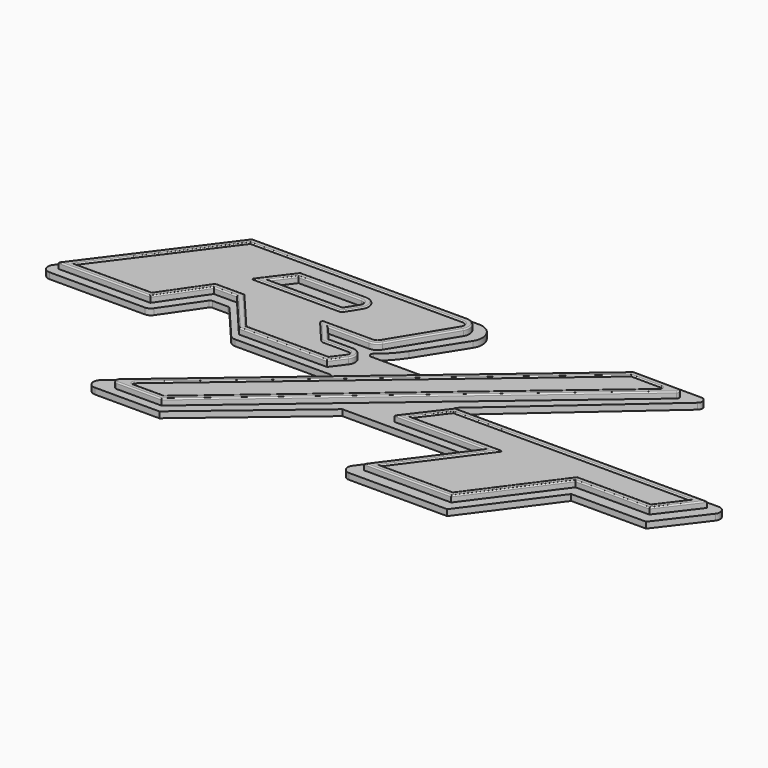
from build123d import *

# Parameters (mm, degrees)
F1_DEPTH = 2.54
F3_DEPTH = 2.54
F5_DEPTH = 2.54
F9_DEPTH = 0.508
F7_R     = 0.50799


# Not quite as in the source:
# - a fillet or chamfer is up to 0.001 mm smaller than in the source, because OpenCascade refuses the exact size


with BuildPart() as f1:
    # F0 (on Top) → F1 (new body)
    with BuildSketch(Plane.XY):
        with BuildLine():
            ThreePointArc((-245.2867057585, 196.0372725906), (-245.8553406914, 195.9028580401), (-246.303608996, 195.5280667845))
            Line((-246.303608996, 195.5280667845), (-286.1584039652, 142.2568005721))
            ThreePointArc((-286.1584039652, 142.2568005721), (-286.4332926298, 139.1776112706), (-283.8030790316, 137.5531276726))
            Line((-283.8030790316, 137.5531276726), (-244.1552884223, 137.5531276726))
            ThreePointArc((-244.1552884223, 137.5531276726), (-242.676229187, 137.9186777658), (-241.5377496314, 138.9311536388))
            Line((-241.5377496314, 138.9311536388), (-230.9500368786, 154.3536073393))
            ThreePointArc((-230.9500368786, 154.3536073393), (-230.4946450563, 154.7585976885), (-229.9030213622, 154.9048177258))
            Line((-229.9030213622, 154.9048177258), (-223.4319893817, 154.9048177258))
            ThreePointArc((-223.4319893817, 154.9048177258), (-222.8981310818, 154.7871611276), (-222.463189241, 154.4559914512))
            Line((-222.463189241, 154.4559914512), (-209.7825220275, 139.4956586958))
            ThreePointArc((-209.7825220275, 139.4956586958), (-208.6951674254, 138.6677345048), (-207.3605216756, 138.3735930092))
            Line((-207.3605216756, 138.3735930092), (-167.7892972517, 138.3735930092))
            ThreePointArc((-167.7892972517, 138.3735930092), (-166.9553293934, 137.7925193173), (-167.2115680195, 136.8089082201))
            Line((-167.2115680195, 136.8089082201), (-223.5524593467, 88.6358837388))
            ThreePointArc((-223.5524593467, 88.6358837388), (-224.401761015, 85.3757095864), (-221.6375786431, 83.4497436876))
            Line((-221.6375786431, 83.4497436876), (-194.8649699805, 83.4497436876))
            Line((-194.8649699805, 83.4497436876), (-149.4059527633, 121.7579135561))
            Line((-149.4059527633, 121.7579135561), (-100.5507462578, 121.7579135561))
            Line((-100.5507462578, 121.7579135561), (-121.9878317389, 92.7682602457))
            ThreePointArc((-121.9878317389, 92.7682602457), (-122.2464609413, 89.7274503693), (-119.6477423423, 88.1274268031))
            Line((-119.6477423423, 88.1274268031), (-78.8742303848, 88.1274268031))
            Line((-78.8742303848, 88.1274268031), (-54.1144270955, 121.6104352103))
            Line((-54.1144270955, 121.6104352103), (-22.9366910897, 121.6104352103))
            Line((-22.9366910897, 121.6104352103), (-8.9016964649, 140.0485662822))
            ThreePointArc((-8.9016964649, 140.0485662822), (-8.6207642896, 142.9884064855), (-11.130164208, 144.5454855965))
            Line((-11.130164208, 144.5454855965), (-120.6925099216, 144.5454855965))
            ThreePointArc((-120.6925099216, 144.5454855965), (-121.2867775914, 144.9567202359), (-121.1113336048, 145.6577818592))
            Line((-121.1113336048, 145.6577818592), (-62.1562381195, 197.3904103448))
            ThreePointArc((-62.1562381195, 197.3904103448), (-61.583083752, 199.680694207), (-63.5244846344, 201.0241482302))
            Line((-63.5244846344, 201.0241482302), (-91.5325754885, 201.0241482302))
            Line((-91.5325754885, 201.0241482302), (-144.0581907195, 156.390979886))
            Line((-144.0581907195, 156.390979886), (-165.1567965746, 156.390979886))
            ThreePointArc((-165.1567965746, 156.390979886), (-166.2861296508, 157.2759629471), (-165.8412963152, 158.6400419474))
            ThreePointArc((-165.8412963152, 158.6400419474), (-161.5040417608, 162.5655921163), (-157.946344878, 167.2093528863))
            Line((-157.946344878, 167.2093528863), (-146.2688178366, 185.7109197082))
            ThreePointArc((-146.2688178366, 185.7109197082), (-146.0663995706, 192.5553078333), (-151.9623764525, 196.0372725906))
            Line((-151.9623764525, 196.0372725906), (-245.2867057585, 196.0372725906))
        make_face()
    extrude(amount=F1_DEPTH)

    # F2 (on face) → F3 (join)
    with BuildSketch(Plane.XY.offset(2.54)):
        with BuildLine():
            Line((-75.6383077882, 195.1749867248), (-88.1063342094, 195.2720095674))
            Line((-88.1063342094, 195.2720095674), (-211.0118440568, 90.8230394157))
            ThreePointArc((-211.0118440568, 90.8230394157), (-211.2321021719, 89.9853005359), (-210.5217670945, 89.4895746581))
            Line((-210.5217670945, 89.4895746581), (-197.7361927904, 89.4895746581))
            Line((-197.7361927904, 89.4895746581), (-75.1047645055, 193.7056216727))
            ThreePointArc((-75.1047645055, 193.7056216727), (-74.860941222, 194.6257070651), (-75.6383077882, 195.1749867248))
        make_face()
        Polygon((-18.5225492173, 139.0465293437), (-117.1023442206, 139.0465293437), (-125.6702630111, 127.7906354944), (-87.9282544571, 127.7906354944), (-112.1474074595, 95.0387555978), (-82.0121606334, 95.0387555978), (-57.1953153693, 128.5989026195), (-26.475219927, 128.5989026195), align=None)
        with BuildLine():
            Line((-154.6691002865, 190.8006613512), (-242.8746338045, 190.8006613512))
            Line((-242.8746338045, 190.8006613512), (-278.1461511696, 143.655558918))
            Line((-278.1461511696, 143.655558918), (-246.0618317127, 143.655558918))
            Line((-246.0618317127, 143.655558918), (-233.8889765025, 161.3869897064))
            Line((-233.8889765025, 161.3869897064), (-221.8132032306, 161.3869897064))
            Line((-221.8132032306, 161.3869897064), (-207.2979211807, 144.2622244358))
            Line((-207.2979211807, 144.2622244358), (-173.0524588328, 144.2622244358))
            Line((-173.0524588328, 144.2622244358), (-169.4335754667, 149.0993462762))
            ThreePointArc((-169.4335754667, 149.0993462762), (-169.2980659943, 150.6172674254), (-170.5946594988, 151.4180749655))
            Line((-170.5946594988, 151.4180749655), (-180.6847838701, 151.4180749655))
            ThreePointArc((-180.6847838701, 151.4180749655), (-181.7775167216, 151.6589014734), (-182.6677814942, 152.3367592212))
            Line((-182.6677814942, 152.3367592212), (-190.4167001347, 161.4787388509))
            ThreePointArc((-190.4167001347, 161.4787388509), (-190.5341831318, 162.3460723754), (-189.7965872333, 162.8172644678))
            Line((-189.7965872333, 162.8172644678), (-169.2928134558, 162.8172644678))
            ThreePointArc((-169.2928134558, 162.8172644678), (-168.2285718133, 163.0956607735), (-167.4369771006, 163.8595276385))
            Line((-167.4369771006, 163.8595276385), (-152.9175816859, 187.6819366499))
            ThreePointArc((-152.9175816859, 187.6819366499), (-152.8806469623, 189.7538804922), (-154.6691002865, 190.8006613512))
        make_face()
        with BuildLine():
            Line((-226.7749905586, 171.6903150082), (-217.0877456665, 184.534072876))
            Line((-217.0877456665, 184.534072876), (-189.6498650312, 184.534072876))
            ThreePointArc((-189.6498650312, 184.534072876), (-185.7910307303, 182.2551757043), (-185.9235106507, 177.7756195264))
            Line((-185.9235106507, 177.7756195264), (-189.3198400657, 172.3945644967))
            ThreePointArc((-189.3198400657, 172.3945644967), (-189.8678435628, 171.8780436065), (-190.5971306368, 171.6903150082))
            Line((-190.5971306368, 171.6903150082), (-226.7749905586, 171.6903150082))
        make_face(mode=Mode.SUBTRACT)
    extrude(amount=F3_DEPTH)

    # F4 (on face) → F5 (join)
    with BuildSketch(Plane.XY.offset(2.54)):
        with BuildLine():
            Line((-70.206199124, 197.5622259258), (-88.9910170645, 197.7084043484))
            Line((-88.9910170645, 197.7084043484), (-216.3343642699, 89.4880203493))
            ThreePointArc((-216.3343642699, 89.4880203493), (-216.7353953667, 87.962721989), (-215.4420652433, 87.0601377988))
            Line((-215.4420652433, 87.0601377988), (-196.8433225219, 87.0601377988))
            Line((-196.8433225219, 87.0601377988), (-69.4065238131, 195.3599398264))
            ThreePointArc((-69.4065238131, 195.3599398264), (-69.0410811838, 196.7389649142), (-70.206199124, 197.5622259258))
        make_face()
        Polygon((-118.3068796381, 141.4772123098), (-130.5752409768, 125.3599525283), (-92.748751834, 125.3599525283), (-116.9679048364, 92.6080726317), (-80.7865153898, 92.6080726317), (-55.9696701257, 126.1682196534), (-25.2706845095, 126.1682196534), (-13.6175712516, 141.4772123098), align=None)
        with BuildLine():
            Line((-154.6691002865, 193.2390613512), (-244.0956422463, 193.2390613512))
            Line((-244.0956422463, 193.2390613512), (-283.0157281162, 141.217158918))
            Line((-283.0157281162, 141.217158918), (-244.7781149145, 141.217158918))
            Line((-244.7781149145, 141.217158918), (-232.6052597042, 158.9485897064))
            Line((-232.6052597042, 158.9485897064), (-222.9428665553, 158.9485897064))
            Line((-222.9428665553, 158.9485897064), (-208.4275845055, 141.8238244358))
            Line((-208.4275845055, 141.8238244358), (-171.831450391, 141.8238244358))
            Line((-171.831450391, 141.8238244358), (-167.4811212506, 147.638621424))
            ThreePointArc((-167.4811212506, 147.638621424), (-167.1177419312, 151.7090464965), (-170.5946594988, 153.8564749655))
            Line((-170.5946594988, 153.8564749655), (-180.6847838701, 153.8564749655))
            ThreePointArc((-180.6847838701, 153.8564749655), (-180.7525087857, 153.8714008048), (-180.807685224, 153.9134127739))
            Line((-180.807685224, 153.9134127739), (-186.2879270512, 160.3788644678))
            Line((-186.2879270512, 160.3788644678), (-169.2928134558, 160.3788644678))
            ThreePointArc((-169.2928134558, 160.3788644678), (-167.0345504492, 160.9696063194), (-165.3548294304, 162.5904903501))
            Line((-165.3548294304, 162.5904903501), (-150.8354340157, 186.4128993614))
            ThreePointArc((-150.8354340157, 186.4128993614), (-150.7545925081, 190.9479018563), (-154.6691002865, 193.2390613512))
        make_face()
        with BuildLine():
            Line((-221.8816466958, 174.1287150082), (-215.872667649, 182.095672876))
            Line((-215.872667649, 182.095672876), (-189.6498650312, 182.095672876))
            ThreePointArc((-189.6498650312, 182.095672876), (-187.9263663476, 181.0778327799), (-187.9855367992, 179.0770966575))
            Line((-187.9855367992, 179.0770966575), (-191.1087782565, 174.1287150082))
            Line((-191.1087782565, 174.1287150082), (-221.8816466958, 174.1287150082))
        make_face(mode=Mode.SUBTRACT)
    extrude(amount=F5_DEPTH)

    # F6 (on face) → F9 (cut)
    with BuildSketch(Plane.XY.offset(5.08)):
        with BuildLine():
            ThreePointArc((-190.4167001347, 161.4787388509), (-190.5341831318, 162.3460723754), (-189.7965872333, 162.8172644678))
            Line((-189.7965872333, 162.8172644678), (-169.2928134558, 162.8172644678))
            ThreePointArc((-169.2928134558, 162.8172644678), (-168.2285718133, 163.0956607735), (-167.4369771006, 163.8595276385))
            Line((-167.4369771006, 163.8595276385), (-152.9175816859, 187.6819366499))
            ThreePointArc((-152.9175816859, 187.6819366499), (-152.8806469623, 189.7538804922), (-154.6691002865, 190.8006613512))
            Line((-154.6691002865, 190.8006613512), (-242.8746338045, 190.8006613512))
            Line((-242.8746338045, 190.8006613512), (-278.1461511696, 143.655558918))
            Line((-278.1461511696, 143.655558918), (-246.0618317127, 143.655558918))
            Line((-246.0618317127, 143.655558918), (-233.8889765025, 161.3869897064))
            Line((-233.8889765025, 161.3869897064), (-221.8132032306, 161.3869897064))
            Line((-221.8132032306, 161.3869897064), (-207.2979211807, 144.2622244358))
            Line((-207.2979211807, 144.2622244358), (-173.0524588328, 144.2622244358))
            Line((-173.0524588328, 144.2622244358), (-169.4335754667, 149.0993462762))
            ThreePointArc((-169.4335754667, 149.0993462762), (-169.2980659943, 150.6172674254), (-170.5946594988, 151.4180749655))
            Line((-170.5946594988, 151.4180749655), (-180.6847838701, 151.4180749655))
            ThreePointArc((-180.6847838701, 151.4180749655), (-181.7775167216, 151.6589014734), (-182.6677814942, 152.3367592212))
            Line((-182.6677814942, 152.3367592212), (-190.4167001347, 161.4787388509))
        make_face()
        with BuildLine():
            Line((-226.7749905586, 171.6903150082), (-217.0877456665, 184.534072876))
            Line((-217.0877456665, 184.534072876), (-189.6498650312, 184.534072876))
            ThreePointArc((-189.6498650312, 184.534072876), (-185.7910307303, 182.2551757043), (-185.9235106507, 177.7756195264))
            Line((-185.9235106507, 177.7756195264), (-189.3198400657, 172.3945644967))
            ThreePointArc((-189.3198400657, 172.3945644967), (-189.8678435628, 171.8780436065), (-190.5971306368, 171.6903150082))
            Line((-190.5971306368, 171.6903150082), (-226.7749905586, 171.6903150082))
        make_face(mode=Mode.SUBTRACT)
        with BuildLine():
            Line((-197.7361927904, 89.4895746581), (-75.1047645055, 193.7056216727))
            ThreePointArc((-75.1047645055, 193.7056216727), (-74.860941222, 194.6257070651), (-75.6383077882, 195.1749867248))
            Line((-75.6383077882, 195.1749867248), (-88.1063342094, 195.2720095674))
            Line((-88.1063342094, 195.2720095674), (-211.0118440568, 90.8230394157))
            ThreePointArc((-211.0118440568, 90.8230394157), (-211.2321021719, 89.9853005359), (-210.5217670945, 89.4895746581))
            Line((-210.5217670945, 89.4895746581), (-197.7361927904, 89.4895746581))
        make_face()
        Polygon((-18.5225492173, 139.0465293437), (-117.1023442206, 139.0465293437), (-125.6702630111, 127.7906354944), (-87.9282544571, 127.7906354944), (-112.1474074595, 95.0387555978), (-82.0121606334, 95.0387555978), (-57.1953153693, 128.5989026195), (-26.475219927, 128.5989026195), align=None)
    extrude(amount=-F9_DEPTH, mode=Mode.SUBTRACT)

    # F7 (radius 0.508 in the source; OpenCascade refuses exactly that, so slightly less here)
    f7_edges = [f1.edges().sort_by_distance(p)[0] for p in [
        (-150.754593, 190.947902, 5.08),
        (-158.095132, 174.501695, 5.08),
        (-199.382371, 193.239061, 5.08),
        (-167.03455, 160.969606, 5.08),
        (-263.555685, 167.22811, 5.08),
        (-177.79037, 160.378864, 5.08),
        (-263.896922, 141.217159, 5.08),
        (-183.547806, 157.146139, 5.08),
        (-238.691687, 150.082874, 5.08),
        (-180.752509, 153.871401, 5.08),
        (-227.774063, 158.94859, 5.08),
        (-175.639722, 153.856475, 5.08),
        (-215.685226, 150.386207, 5.08),
        (-167.117742, 151.709046, 5.08),
        (-190.129517, 141.823824, 5.08),
        (-169.656286, 144.731223, 5.08),
        (-171.243017, 146.680785, 5.08),
        (-169.298066, 150.617267, 5.08),
        (-175.639722, 151.418075, 5.08),
        (-181.777517, 151.658901, 5.08),
        (-186.542241, 156.907749, 5.08),
        (-190.534183, 162.346072, 5.08),
        (-179.5447, 162.817264, 5.08),
        (-168.228572, 163.095661, 5.08),
        (-160.177279, 175.770732, 5.08),
        (-152.880647, 189.75388, 5.08),
        (-198.771867, 190.800661, 5.08),
        (-260.510392, 167.22811, 5.08),
        (-262.103991, 143.655559, 5.08),
        (-239.975404, 152.521274, 5.08),
        (-227.85109, 161.38699, 5.08),
        (-214.555562, 152.824607, 5.08),
        (-190.17519, 144.262224, 5.08),
        (-69.041081, 196.738965, 5.08),
        (-133.124923, 141.210039, 5.08),
        (-79.598608, 197.635315, 5.08),
        (-206.142694, 87.060138, 5.08),
        (-152.662691, 143.598212, 5.08),
        (-216.735395, 87.962722, 5.08),
        (-136.420479, 141.597598, 5.08),
        (-74.860941, 194.625707, 5.08),
        (-81.872321, 195.223498, 5.08),
        (-149.559089, 143.047524, 5.08),
        (-211.232102, 89.985301, 5.08),
        (-204.12898, 89.489575, 5.08),
        (-65.962225, 141.477212, 5.08),
        (-19.444128, 133.822716, 5.08),
        (-124.44106, 133.418582, 5.08),
        (-40.620177, 126.16822, 5.08),
        (-111.661996, 125.359953, 5.08),
        (-68.378093, 109.388146, 5.08),
        (-104.858328, 108.984013, 5.08),
        (-98.87721, 92.608073, 5.08),
        (-22.498885, 133.822716, 5.08),
        (-67.812447, 139.046529, 5.08),
        (-121.386304, 133.418582, 5.08),
        (-106.799259, 127.790635, 5.08),
        (-100.037831, 111.414696, 5.08),
        (-97.079784, 95.038756, 5.08),
        (-69.603738, 111.818829, 5.08),
        (-41.835268, 128.598903, 5.08),
        (-221.931368, 178.112194, 5.08),
        (-203.368805, 184.534073, 5.08),
        (-185.791031, 182.255176, 5.08),
        (-187.621675, 175.085092, 5.08),
        (-189.867844, 171.878044, 5.08),
        (-208.686061, 171.690315, 5.08),
        (-218.877157, 178.112194, 5.08),
        (-206.495212, 174.128715, 5.08),
        (-202.761266, 182.095673, 5.08),
        (-189.547158, 176.602906, 5.08),
        (-187.926366, 181.077833, 5.08),
    ]]
    fillet(f7_edges, radius=F7_R)


solid = f1.part
